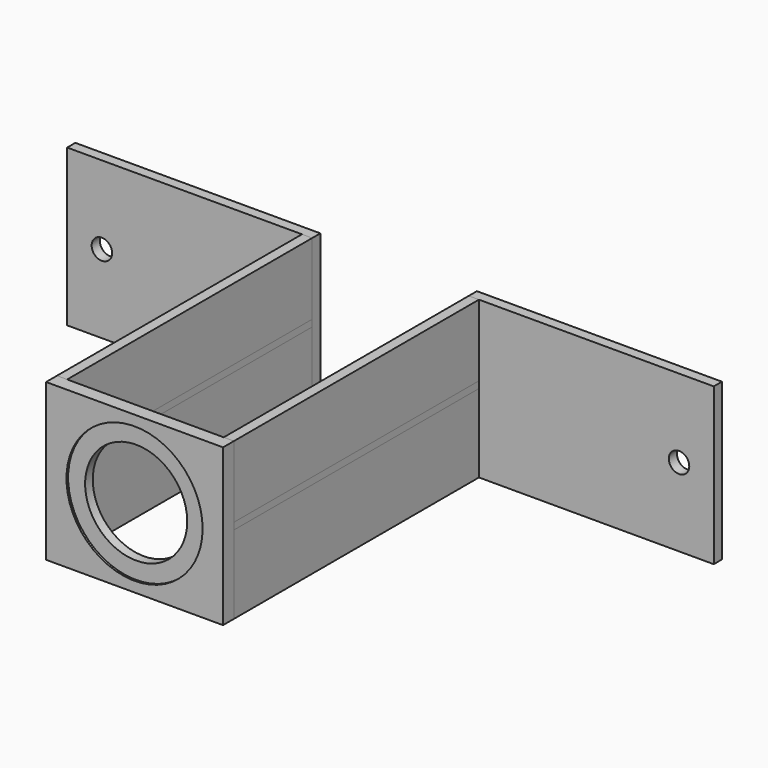
from build123d import *

# Parameters (mm, degrees)
F0_W      = 36
F0_H      = 23
F0_R      = 1.5
F1_DEPTH  = 1.5
F2_W      = 1.5
F2_H      = 45
F3_DEPTH  = 11.5
F4_DEPTH  = 1
F6_DEPTH  = 2
F7_R      = 10
F7_R_2    = 7.5
F8_DEPTH  = 0.3
F9_DEPTH  = 2.2
F10_R     = 10
F10_R_2   = 7.5
F11_DEPTH = 0.3


# Not quite as in the source:
# - ends of sketch curves that miss each other by under 0.0002 mm in the source are joined


with BuildPart() as f1:
    # F0 (on Front) → F1 (new body)
    with BuildSketch(Plane.XZ):
        with Locations((-29.5, 0)):
            Rectangle(F0_W, F0_H)
        with Locations((-42.4, 0)):
            Circle(F0_R, mode=Mode.SUBTRACT)
    extrude(amount=F1_DEPTH)


with BuildPart() as f1b:
    # F0 (on Front) → F1, piece 2 (new body)
    with BuildSketch(Plane.XZ):
        with Locations((29.5, 0)):
            Rectangle(F0_W, F0_H)
        with Locations((42.4, 0)):
            Circle(F0_R, mode=Mode.SUBTRACT)
    extrude(amount=F1_DEPTH)


with BuildPart() as f3:
    # F2 (on Top) → F3 (new body, symmetric)
    with BuildSketch(Plane.XY):
        with Locations((12.2499515936, -24.0000421973)):
            Rectangle(F2_W, F2_H)
    extrude(amount=F3_DEPTH, both=True)


with BuildPart() as f3b:
    # F2 (on Top) → F3, piece 2 (new body, symmetric)
    with BuildSketch(Plane.XY):
        with Locations((-12.2500094585, -24.0000799907)):
            Rectangle(F2_W, F2_H)
    extrude(amount=F3_DEPTH, both=True)


with BuildPart() as f4:
    # F2 (on Top) → F4 (new body)
    with BuildSketch(Plane.XY):
        with Locations((-12.2500094585, -24.0000799907)):
            Rectangle(F2_W, F2_H)
    extrude(amount=F4_DEPTH)


with BuildPart() as f4b:
    # F2 (on Top) → F4, piece 2 (new body)
    with BuildSketch(Plane.XY):
        with Locations((12.2499515936, -24.0000421973)):
            Rectangle(F2_W, F2_H)
    extrude(amount=F4_DEPTH)


with BuildPart() as f6:
    # F5 (on face) → F6 (new body)
    with BuildSketch(Plane.XZ.offset(46.5000421973)):
        Polygon((12.9999515936, -11.5000382066), (12.9999515936, 11.5), (11.4999515936, 11.5), (11.4999515936, -11.5), align=None)
        Polygon((11.4999515936, -11.5), (11.4999515936, 11.5), (-12.9975853488, 11.5), (-12.9975853488, -11.5000382066), align=None)
    extrude(amount=F6_DEPTH)

    # F7 (on face) → F8 (cut)
    with BuildSketch(Plane.XZ.offset(48.5000421973)):
        Circle(F7_R)
        Circle(F7_R_2, mode=Mode.SUBTRACT)
    extrude(amount=-F8_DEPTH, mode=Mode.SUBTRACT)

    # F9 (cut): a face of the model
    f9_faces = [f6.faces().sort_by_distance(p)[0] for p in [
        (0, -48.5000421973, 0),
    ]]
    extrude(f9_faces, amount=-F9_DEPTH, mode=Mode.SUBTRACT)

    # F10 (on face) → F11 (cut)
    with BuildSketch(Plane(origin=(0, -46.5000421973, 0), x_dir=(-1, 0, 0), z_dir=(0, 1, 0))):
        with Locations((0, 0.2298883747)):
            Circle(F10_R)
        Circle(F10_R_2, mode=Mode.SUBTRACT)
    extrude(amount=-F11_DEPTH, mode=Mode.SUBTRACT)


solid = Compound([f1.part, f1b.part, f3.part, f3b.part, f4.part, f4b.part, f6.part])
